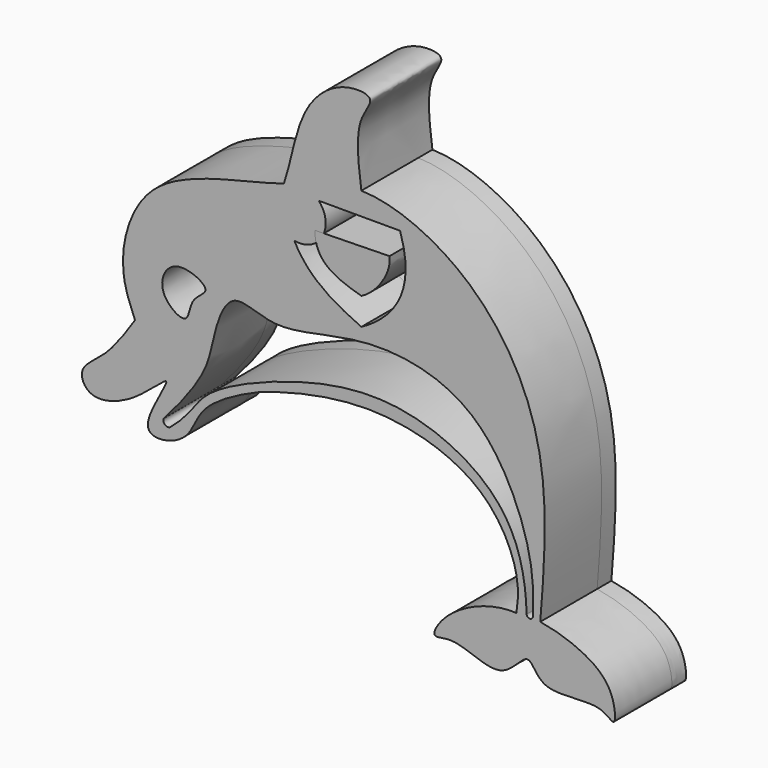
from build123d import *

# Parameters (mm, degrees)
F1_DEPTH = 2
F5_DEPTH = 10
F6_R     = 2.9226777264
F7_DEPTH = 10


# Not quite as in the source:
# - a feature of the source that left no trace in its solid (it failed there, or was rolled back) is left out


with BuildPart() as f1:
    # F0 (on Front) → F1 (new body)
    with BuildSketch(Plane.XZ):
        with BuildLine():
            add(Edge.make_bspline(
                [(-25.4752909133, -7.6226384082), (-26.1474454794, -6.0257169075), (-27.6328894573, -2.4574095527), (-24.6240452229, 8.324114137), (-13.6020689967, 9.8657928331), (-8.9893052775, 11.2778379539), (-8.7112760799, 11.3657612806)],
                knots=[0, 0, 0, 0, 0.09619522, 0.2228627615, 0.3812812799, 0.3916577764, 0.3916577764, 0.3916577764, 0.3916577764], degree=3))
            add(Edge.make_bspline(
                [(17.4490734935, -22.6735323523), (17.6184843518, -21.5208863246), (17.9014397151, -18.6492794271), (14.1409068293, -10.4449029024), (0.9364651731, -6.5775299665), (-10.4499868797, -9.7410841929), (-12.9229059082, -10.769885563), (-18.302854281, -13.5735615064), (-19.1226009113, -17.4328358412), (-22.5628593483, -18.8177496782), (-25.1440149682, -17.8289423021), (-20.056055785, -10.2018009579), (-25.6082423385, -16.0296131413), (-30.6338712907, -17.3819434747), (-32.0501239108, -14.2293860564), (-28.6216951915, -12.3200736245), (-26.621485389, -9.3369011161), (-25.4752909133, -7.6226384082)],
                knots=[0, 0, 0, 0, 0.0585716887, 0.1437279624, 0.2542500472, 0.3549075489, 0.4057900144, 0.4764797276, 0.534787487, 0.5894467381, 0.6281369999, 0.6974719038, 0.7607683636, 0.8290857956, 0.8723976286, 0.9271372009, 1, 1, 1, 1], degree=3))
            add(Edge.make_bspline(
                [(20.1342925429, -22.6735323523), (21.8137129432, -22.9389697516), (25.1403629861, -23.9711834635), (28.4299265216, -26.5482573008), (28.7643629279, -30.8558421047), (26.7889548575, -28.1575658974), (20.1223197883, -30.0736915306), (18.8744382455, -25.4250533032), (15.9065710136, -30.5693085112), (10.6625417605, -27.0727168364), (7.5710867138, -28.5263464708), (9.526934773, -24.7098479997), (14.5109416263, -22.5015593339), (17.4490734935, -22.6735323523)],
                knots=[0, 0, 0, 0, 0.1050620871, 0.2007285629, 0.2767396193, 0.3381884123, 0.4539107022, 0.5286066305, 0.6158006039, 0.7253352098, 0.7913814677, 0.865443081, 1, 1, 1, 1], degree=3))
            add(Edge.make_bspline(
                [(0, 13.4910019115), (3.7782424934, 13.4165937552), (13.4195566651, 9.2563857307), (21.5608771506, -4.7801001723), (20.6169119806, -16.5972898916), (20.1342925429, -22.6735323523)],
                knots=[0.5117289148, 0.5117289148, 0.5117289148, 0.5117289148, 0.6620421525, 0.8248838893, 1, 1, 1, 1], degree=3))
            add(Edge.make_bspline(
                [(-8.7112760799, 11.3657612806), (-5.4940743828, 12.3831618924), (-3.0180833334, 13.5504396042), (0, 13.4910019115)],
                knots=[0.3916577764, 0.3916577764, 0.3916577764, 0.3916577764, 0.5117289148, 0.5117289148, 0.5117289148, 0.5117289148], degree=3))
        make_face()
        with BuildLine():
            add(Edge.make_bspline(
                [(-21.4838143438, -16.9164761901), (-20.8433505346, -16.4160758348), (-19.0086116044, -14.5208074776), (-17.199070095, -11.3112198959), (-4.1982117704, -6.1412196867), (6.7943031443, -6.3054430606), (16.7405120951, -11.8902969647), (18.492605338, -18.480320762), (18.5979679227, -22.4138069898)],
                knots=[0, 0, 0, 0, 0.1039074622, 0.2153773153, 0.4280713673, 0.626076108, 0.8124990775, 1, 1, 1, 1], degree=3))
            ThreePointArc((-21.4838143438, -16.9164761901), (-22.1032394124, -16.8846246549), (-22.2294498235, -16.2773579359))
            add(Edge.make_bspline(
                [(-22.2294498235, -16.2773579359), (-21.2777016749, -15.2659020368), (-17.1155222223, -10.3500456153), (-16.7573319358, -6.0480046613), (-14.6554102705, -0.7111884334), (-9.4991498153, -4.0054150901), (0.1124510584, -0.3428046468), (13.86715981, -2.7164947488), (19.5430710176, -16.1368977538), (19.3418966312, -20.5825998672), (19.3042379561, -22.4138069898)],
                knots=[0, 0, 0, 0, 0.1227667244, 0.2246070138, 0.3180037771, 0.4139087075, 0.558102917, 0.721908091, 0.8874903385, 1, 1, 1, 1], degree=3))
            ThreePointArc((19.3042379561, -22.4138069898), (18.9511029394, -22.750498355), (18.5979679227, -22.4138069898))
        make_face(mode=Mode.SUBTRACT)
        with BuildLine():
            add(Edge.make_bspline(
                [(-19.8578462005, -5.6317406707), (-20.4743685031, -5.8837360132), (-23.3455691815, -3.928385761), (-21.3541919898, 0.3953469963), (-16.2293425802, -1.9901837601), (-19.4372398584, -3.2173104238), (-19.3228946234, -5.4130862841), (-19.8578462005, -5.6317406707)],
                knots=[0, 0, 0, 0, 0.2086836247, 0.4264173541, 0.6477830052, 0.8189268521, 1, 1, 1, 1], degree=3))
        make_face(mode=Mode.SUBTRACT)
        with BuildLine():
            ThreePointArc((-8.0441749995, 7.26742557), (-8.9116094438, 9.3592918369), (-7.2894585319, 10.9394732863))
            ThreePointArc((-7.2894585319, 10.9394732863), (-6.9351789483, 10.970819341), (-6.5808993647, 10.9394732863))
            Line((-6.5808993647, 10.9394732863), (4.3582133949, 10.9394732863))
            add(Edge.make_bspline(
                [(4.3582133949, 10.9394732863), (5.8316430077, 6.4374315552), (4.8221717589, 2.6519128587), (0, 0)],
                knots=[0, 0, 0, 0, 11.7756570847, 11.7756570847, 11.7756570847, 11.7756570847], degree=3))
            add(Edge.make_bspline(
                [(0, 0), (-3.3797856886, 1.5162572963), (-6.6561518577, 3.3557229092), (-8.0441749995, 7.26742557)],
                knots=[0, 0, 0, 0, 10.8408590913, 10.8408590913, 10.8408590913, 10.8408590913], degree=3))
        make_face(mode=Mode.SUBTRACT)
    extrude(amount=F1_DEPTH)

    # F0 (on Front) → F5 (join)
    with BuildSketch(Plane.XZ):
        with BuildLine():
            add(Edge.make_bspline(
                [(-25.4752909133, -7.6226384082), (-26.1474454794, -6.0257169075), (-27.6328894573, -2.4574095527), (-24.6240452229, 8.324114137), (-13.6020689967, 9.8657928331), (-8.9893052775, 11.2778379539), (-8.7112760799, 11.3657612806)],
                knots=[0, 0, 0, 0, 0.09619522, 0.2228627615, 0.3812812799, 0.3916577764, 0.3916577764, 0.3916577764, 0.3916577764], degree=3))
            add(Edge.make_bspline(
                [(17.4490734935, -22.6735323523), (17.6184843518, -21.5208863246), (17.9014397151, -18.6492794271), (14.1409068293, -10.4449029024), (0.9364651731, -6.5775299665), (-10.4499868797, -9.7410841929), (-12.9229059082, -10.769885563), (-18.302854281, -13.5735615064), (-19.1226009113, -17.4328358412), (-22.5628593483, -18.8177496782), (-25.1440149682, -17.8289423021), (-20.056055785, -10.2018009579), (-25.6082423385, -16.0296131413), (-30.6338712907, -17.3819434747), (-32.0501239108, -14.2293860564), (-28.6216951915, -12.3200736245), (-26.621485389, -9.3369011161), (-25.4752909133, -7.6226384082)],
                knots=[0, 0, 0, 0, 0.0585716887, 0.1437279624, 0.2542500472, 0.3549075489, 0.4057900144, 0.4764797276, 0.534787487, 0.5894467381, 0.6281369999, 0.6974719038, 0.7607683636, 0.8290857956, 0.8723976286, 0.9271372009, 1, 1, 1, 1], degree=3))
            add(Edge.make_bspline(
                [(20.1342925429, -22.6735323523), (21.8137129432, -22.9389697516), (25.1403629861, -23.9711834635), (28.4299265216, -26.5482573008), (28.7643629279, -30.8558421047), (26.7889548575, -28.1575658974), (20.1223197883, -30.0736915306), (18.8744382455, -25.4250533032), (15.9065710136, -30.5693085112), (10.6625417605, -27.0727168364), (7.5710867138, -28.5263464708), (9.526934773, -24.7098479997), (14.5109416263, -22.5015593339), (17.4490734935, -22.6735323523)],
                knots=[0, 0, 0, 0, 0.1050620871, 0.2007285629, 0.2767396193, 0.3381884123, 0.4539107022, 0.5286066305, 0.6158006039, 0.7253352098, 0.7913814677, 0.865443081, 1, 1, 1, 1], degree=3))
            add(Edge.make_bspline(
                [(0, 13.4910019115), (3.7782424934, 13.4165937552), (13.4195566651, 9.2563857307), (21.5608771506, -4.7801001723), (20.6169119806, -16.5972898916), (20.1342925429, -22.6735323523)],
                knots=[0.5117289148, 0.5117289148, 0.5117289148, 0.5117289148, 0.6620421525, 0.8248838893, 1, 1, 1, 1], degree=3))
            add(Edge.make_bspline(
                [(-8.7112760799, 11.3657612806), (-5.4940743828, 12.3831618924), (-3.0180833334, 13.5504396042), (0, 13.4910019115)],
                knots=[0.3916577764, 0.3916577764, 0.3916577764, 0.3916577764, 0.5117289148, 0.5117289148, 0.5117289148, 0.5117289148], degree=3))
        make_face()
        with BuildLine():
            add(Edge.make_bspline(
                [(-21.4838143438, -16.9164761901), (-20.8433505346, -16.4160758348), (-19.0086116044, -14.5208074776), (-17.199070095, -11.3112198959), (-4.1982117704, -6.1412196867), (6.7943031443, -6.3054430606), (16.7405120951, -11.8902969647), (18.492605338, -18.480320762), (18.5979679227, -22.4138069898)],
                knots=[0, 0, 0, 0, 0.1039074622, 0.2153773153, 0.4280713673, 0.626076108, 0.8124990775, 1, 1, 1, 1], degree=3))
            ThreePointArc((-21.4838143438, -16.9164761901), (-22.1032394124, -16.8846246549), (-22.2294498235, -16.2773579359))
            add(Edge.make_bspline(
                [(-22.2294498235, -16.2773579359), (-21.2777016749, -15.2659020368), (-17.1155222223, -10.3500456153), (-16.7573319358, -6.0480046613), (-14.6554102705, -0.7111884334), (-9.4991498153, -4.0054150901), (0.1124510584, -0.3428046468), (13.86715981, -2.7164947488), (19.5430710176, -16.1368977538), (19.3418966312, -20.5825998672), (19.3042379561, -22.4138069898)],
                knots=[0, 0, 0, 0, 0.1227667244, 0.2246070138, 0.3180037771, 0.4139087075, 0.558102917, 0.721908091, 0.8874903385, 1, 1, 1, 1], degree=3))
            ThreePointArc((19.3042379561, -22.4138069898), (18.9511029394, -22.750498355), (18.5979679227, -22.4138069898))
        make_face(mode=Mode.SUBTRACT)
        with BuildLine():
            add(Edge.make_bspline(
                [(-19.8578462005, -5.6317406707), (-20.4743685031, -5.8837360132), (-23.3455691815, -3.928385761), (-21.3541919898, 0.3953469963), (-16.2293425802, -1.9901837601), (-19.4372398584, -3.2173104238), (-19.3228946234, -5.4130862841), (-19.8578462005, -5.6317406707)],
                knots=[0, 0, 0, 0, 0.2086836247, 0.4264173541, 0.6477830052, 0.8189268521, 1, 1, 1, 1], degree=3))
        make_face(mode=Mode.SUBTRACT)
        with BuildLine():
            ThreePointArc((-8.0441749995, 7.26742557), (-8.9116094438, 9.3592918369), (-7.2894585319, 10.9394732863))
            ThreePointArc((-7.2894585319, 10.9394732863), (-6.9351789483, 10.970819341), (-6.5808993647, 10.9394732863))
            Line((-6.5808993647, 10.9394732863), (4.3582133949, 10.9394732863))
            add(Edge.make_bspline(
                [(4.3582133949, 10.9394732863), (5.8316430077, 6.4374315552), (4.8221717589, 2.6519128587), (0, 0)],
                knots=[0, 0, 0, 0, 11.7756570847, 11.7756570847, 11.7756570847, 11.7756570847], degree=3))
            add(Edge.make_bspline(
                [(0, 0), (-3.3797856886, 1.5162572963), (-6.6561518577, 3.3557229092), (-8.0441749995, 7.26742557)],
                knots=[0, 0, 0, 0, 10.8408590913, 10.8408590913, 10.8408590913, 10.8408590913], degree=3))
        make_face(mode=Mode.SUBTRACT)
        with BuildLine():
            add(Edge.make_bspline(
                [(-8.7112760799, 11.3657612806), (-7.8834280783, 13.7644339805), (-7.202830405, 19.5379933143), (-2.6027396832, 23.6103456541), (2.004801359, 23.3050711184), (-0.8840128352, 20.315740577), (-0.3346707075, 16.0657270507), (0, 13.4910019115)],
                knots=[0, 0, 0, 0, 0.2550192121, 0.470889692, 0.6217825225, 0.763591342, 1, 1, 1, 1], degree=3))
            add(Edge.make_bspline(
                [(-8.7112760799, 11.3657612806), (-5.4940743828, 12.3831618924), (-3.0180833334, 13.5504396042), (0, 13.4910019115)],
                knots=[0.3916577764, 0.3916577764, 0.3916577764, 0.3916577764, 0.5117289148, 0.5117289148, 0.5117289148, 0.5117289148], degree=3))
        make_face()
    extrude(amount=F5_DEPTH)

    # F6 (on face) → F7 (join)
    with BuildSketch(Plane.XZ):
        with Locations((-6.9351789483, 8.9530758078)):
            Circle(F6_R)
    extrude(amount=F7_DEPTH)


with BuildPart() as f5:
    # F0 (on Front) → F5, piece 2 (new body)
    with BuildSketch(Plane.XZ):
        with BuildLine():
            Line((3.1705347355, 8.0388048664), (-5.232644733, 7.8701786697))
            add(Edge.make_bspline(
                [(-5.232644733, 7.8701786697), (-5.232644733, 4.9679479562), (-3.12741776, 3.9516080444), (0, 3.0683200613)],
                knots=[0, 0, 0, 0, 7.102000915, 7.102000915, 7.102000915, 7.102000915], degree=3))
            add(Edge.make_bspline(
                [(0, 3.0683200613), (1.7372167204, 3.9355796762), (3.4149778968, 6.3458379361), (3.1705347355, 8.0388048664)],
                knots=[0, 0, 0, 0, 5.8955923966, 5.8955923966, 5.8955923966, 5.8955923966], degree=3))
        make_face()
    extrude(amount=F5_DEPTH)


solid = Compound([f1.part, f5.part])
